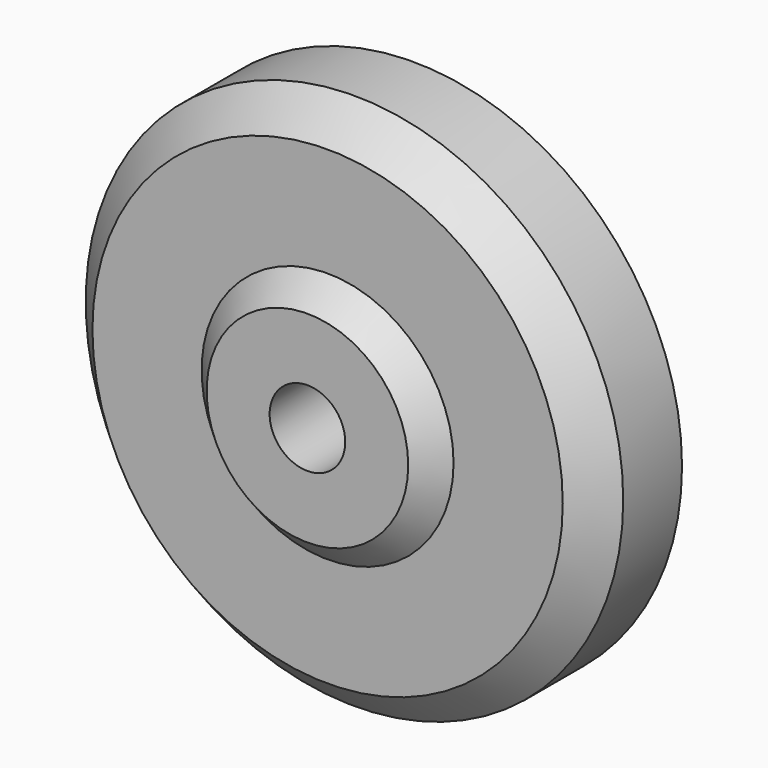
from build123d import *

# Parameters (mm, degrees)
F0_R      = 64
F1_DEPTH  = 25.5
F2_R      = 58
F3_DEPTH  = 1
F4_SIZE   = 8
F5_R      = 30
F6_DEPTH  = 6
F7_SIZE   = 5.99999
F9_R      = 9
F10_DEPTH = 18


# Not quite as in the source:
# - a fillet or chamfer is up to 0.001 mm smaller than in the source, because OpenCascade refuses the exact size


with BuildPart() as f1:
    # F0 (on Front) → F1 (new body)
    with BuildSketch(Plane.XZ):
        Circle(F0_R)
    extrude(amount=F1_DEPTH)

    # F2 (on face) → F3 (cut)
    with BuildSketch(Plane(origin=(0, 0, 0), x_dir=(-1, 0, 0), z_dir=(0, 1, 0))):
        Circle(F2_R)
    extrude(amount=-F3_DEPTH, mode=Mode.SUBTRACT)

    # F4
    f4_edges = [f1.edges().sort_by_distance(p)[0] for p in [
        (-64, -25.5, 0),
    ]]
    chamfer(f4_edges, length=F4_SIZE)

    # F5 (on face) → F6 (join)
    with BuildSketch(Plane.XZ.offset(25.5)):
        Circle(F5_R)
    extrude(amount=F6_DEPTH)

    # F7 (size 6 in the source; OpenCascade refuses exactly that, so slightly less here)
    f7_edges = [f1.edges().sort_by_distance(p)[0] for p in [
        (-30, -31.5, 0),
    ]]
    chamfer(f7_edges, length=F7_SIZE)

    # F9 (on face) → F10 (cut)
    with BuildSketch(Plane.XZ.offset(31.5)):
        Circle(F9_R)
    extrude(amount=-F10_DEPTH, mode=Mode.SUBTRACT)


solid = f1.part
